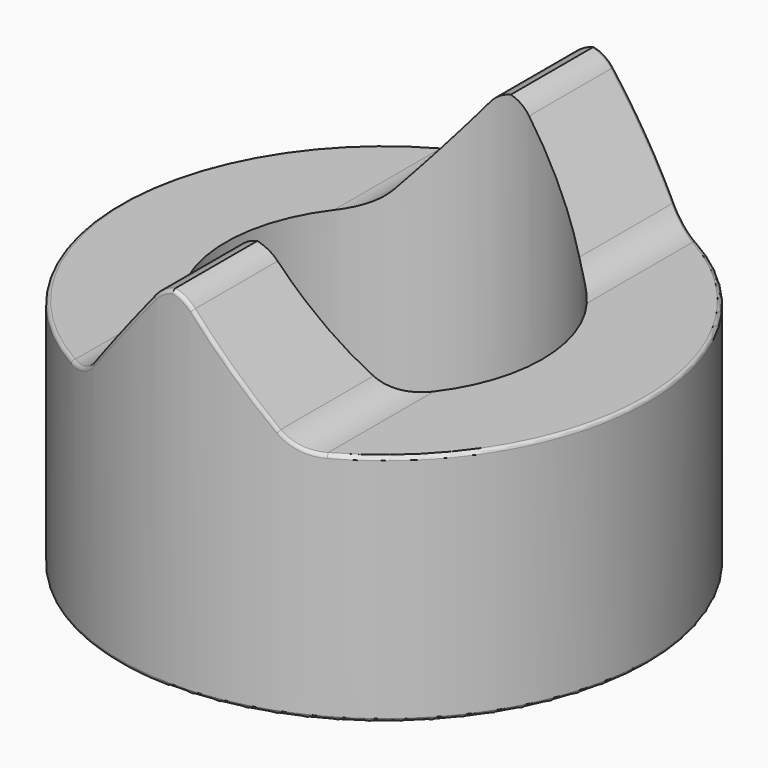
from build123d import *

# Parameters (mm, degrees)
F0_R        = 38.1
F0_R_2      = 22.86
F1_DEPTH    = 50.8
F4_DEPTH    = 83.567
F5_T1_DEPTH = 27.2653813946
F5_T3_DEPTH = 27.2653813946
F6_R        = 0.508


# Not quite as in the source:
# - a fillet or chamfer that OpenCascade refuses, or shapes differently, is made with other operations: its cross-section is extruded or revolved along the edge and cut away or added
# - two fillets or chamfers of one size are made in one step


with BuildPart() as f1:
    # F0 (on Top) → F1 (new body)
    with BuildSketch(Plane.XY):
        Circle(F0_R)
        Circle(F0_R_2, mode=Mode.SUBTRACT)
    extrude(amount=F1_DEPTH)

    # F3 (on offset) → F4 (cut, through all)
    with BuildSketch(Plane.XZ.offset(45.466)):
        with BuildLine():
            Line((-38.1, 50.8), (-38.1, 33.7820982995))
            Line((-38.1, 33.7820982995), (-18.242812226, 33.7820982995))
            ThreePointArc((-18.242812226, 33.7820982995), (-15.5282171859, 34.39158667), (-13.3347289514, 36.1030514433))
            Line((-13.3347289514, 36.1030514433), (-1.2895432809, 50.776192868))
            Line((-1.2895432809, 50.776192868), (-1.27, 50.8))
            Line((-1.27, 50.8), (-38.1, 50.8))
        make_face()
        with BuildLine():
            Line((18.242812226, 33.7820982995), (38.1, 33.7820982995))
            Line((38.1, 33.7820982995), (38.1, 50.8))
            Line((38.1, 50.8), (1.27, 50.8))
            Line((1.27, 50.8), (1.2895432809, 50.776192868))
            Line((1.2895432809, 50.776192868), (13.3347289514, 36.1030514433))
            ThreePointArc((13.3347289514, 36.1030514433), (15.5282171859, 34.39158667), (18.242812226, 33.7820982995))
        make_face()
    extrude(amount=-F4_DEPTH, mode=Mode.SUBTRACT)

    # F5: fillet of radius 5.08 on 4 edges, made by hand

    # F5_s2 → F5_t1 (cut)
    with BuildSketch(Plane.XZ.offset(16.8190705077)):
        with BuildLine():
            ThreePointArc((2.7942168389, 48.943237485), (1.0394262513, 50.3124093036), (-1.1322497808, 50.8))
            Line((-1.1322497808, 50.8), (1.27, 50.8))
            Line((1.27, 50.8), (2.7942168389, 48.943237485))
        make_face()
        with BuildLine():
            ThreePointArc((1.1322497808, 50.8), (-1.0394262513, 50.3124093036), (-2.7942168389, 48.943237485))
            Line((-2.7942168389, 48.943237485), (-1.27, 50.8))
            Line((-1.27, 50.8), (1.1322497808, 50.8))
        make_face()
    extrude(amount=F5_T1_DEPTH, mode=Mode.SUBTRACT)

    # F5_s4 → F5_t3 (cut)
    with BuildSketch(Plane.XZ.offset(-44.0844519023)):
        with BuildLine():
            ThreePointArc((-1.1322497808, 50.8), (1.0394262513, 50.3124093036), (2.7942168389, 48.943237485))
            Line((2.7942168389, 48.943237485), (1.27, 50.8))
            Line((1.27, 50.8), (-1.1322497808, 50.8))
        make_face()
        with BuildLine():
            ThreePointArc((-2.7942168389, 48.943237485), (-1.0394262513, 50.3124093036), (1.1322497808, 50.8))
            Line((1.1322497808, 50.8), (-1.27, 50.8))
            Line((-1.27, 50.8), (-2.7942168389, 48.943237485))
        make_face()
    extrude(amount=F5_T3_DEPTH, mode=Mode.SUBTRACT)

    # F6
    f6_edges = [f1.edges().sort_by_distance(p)[0] for p in [
        (32.761724, 19.449407, 33.782098),
        (32.761724, -19.449407, 33.782098),
        (-38.1, 0, 0),
        (15.502624, -34.803429, 34.403759),
        (8.14656, -37.21886, 42.423148),
        (1.617944, -38.065631, 49.991163),
        (-1.617945, -38.065631, 49.991163),
        (-8.14656, -37.21886, 42.423148),
        (-15.498358, -34.805329, 34.405802),
        (-38.1, 0, 33.782098),
        (-15.498358, 34.805329, 34.405802),
        (-8.14656, 37.21886, 42.423148),
        (-1.617944, 38.065631, 49.991163),
        (1.617945, 38.065631, 49.991163),
        (8.14656, 37.21886, 42.423148),
        (15.502624, 34.803429, 34.403759),
    ]]
    fillet(f6_edges, radius=F6_R)


solid = f1.part
